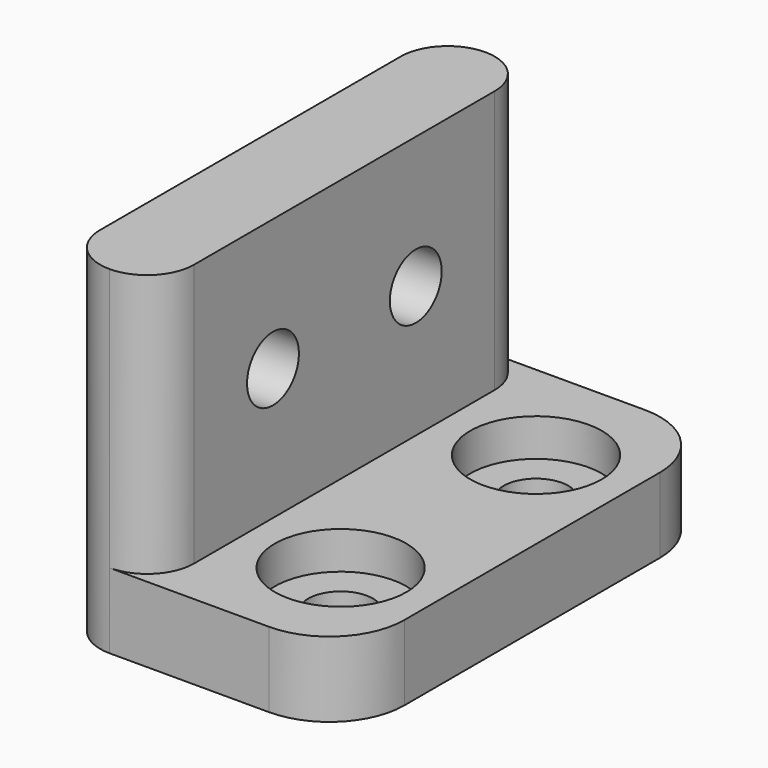
from build123d import *

# Parameters (mm, degrees)
F0_W     = 15
F0_H     = 25
F1_DEPTH = 4
F2_W     = 5
F2_H     = 25
F3_DEPTH = 14
F4_R     = 3.5
F4_R_2   = 1.725
F5_DEPTH = 2
F6_DEPTH = 4
F7_R     = 1.725
F8_DEPTH = 5
F9_R     = 4
F10_R    = 2.49999


# Not quite as in the source:
# - a fillet or chamfer is up to 0.001 mm smaller than in the source, because OpenCascade refuses the exact size


with BuildPart() as f1:
    # F0 (on Top) → F1 (new body)
    with BuildSketch(Plane.XY):
        with Locations((7.5, 12.5)):
            Rectangle(F0_W, F0_H)
    extrude(amount=F1_DEPTH)

    # F2 (on face) → F3 (join)
    with BuildSketch(Plane.XY.offset(4)):
        with Locations((2.5, 12.5)):
            Rectangle(F2_W, F2_H)
    extrude(amount=F3_DEPTH)

    # F4 (on face) → F5 (cut)
    with BuildSketch(Plane.XY.offset(4)):
        with Locations((10, 19)):
            Circle(F4_R)
        with Locations((10, 19)):
            Circle(F4_R_2, mode=Mode.SUBTRACT)
        with Locations((10, 6)):
            Circle(F4_R)
        with Locations((10, 6)):
            Circle(F4_R_2, mode=Mode.SUBTRACT)
    extrude(amount=-F5_DEPTH, mode=Mode.SUBTRACT)

    # F4 (on face) → F6 (cut, through all)
    with BuildSketch(Plane.XY.offset(4)):
        with Locations((10, 19)):
            Circle(F4_R_2)
        with Locations((10, 6)):
            Circle(F4_R_2)
    extrude(amount=-F6_DEPTH, mode=Mode.SUBTRACT)

    # F7 (on face) → F8 (cut, through all)
    with BuildSketch(Plane.YZ.offset(5)):
        with Locations((7.75, 11)):
            Circle(F7_R)
        with Locations((17.25, 11)):
            Circle(F7_R)
    extrude(amount=-F8_DEPTH, mode=Mode.SUBTRACT)

    # F9
    f9_edges = [f1.edges().sort_by_distance(p)[0] for p in [
        (15, 0, 2),
        (15, 25, 2),
    ]]
    fillet(f9_edges, radius=F9_R)

    # F10 (radius 2.5 in the source; OpenCascade refuses exactly that, so slightly less here)
    f10_edges = [f1.edges().sort_by_distance(p)[0] for p in [
        (0, 0, 9),
        (0, 25, 9),
        (5, 25, 11),
        (5, 0, 11),
    ]]
    fillet(f10_edges, radius=F10_R)


solid = f1.part
